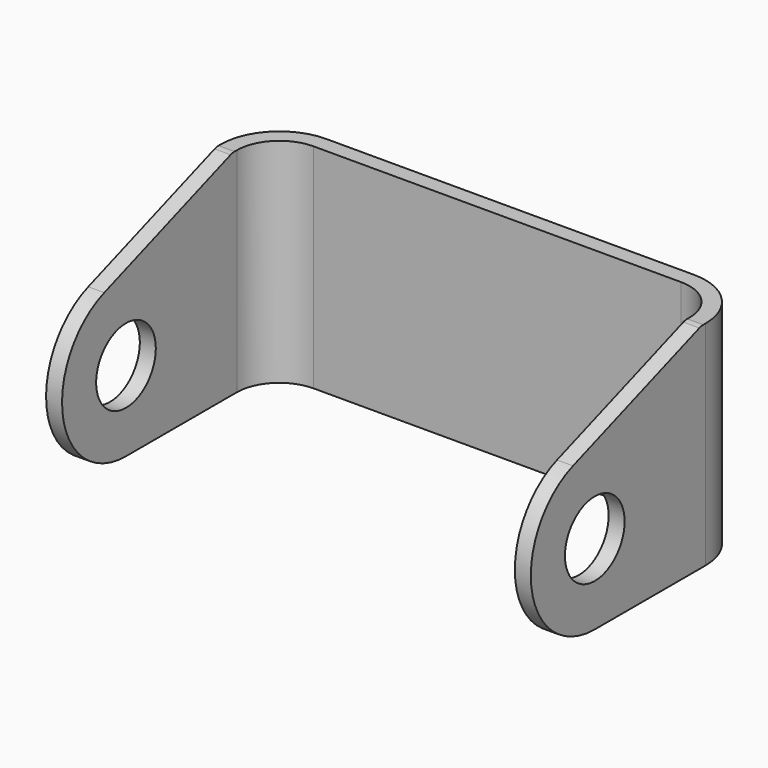
from build123d import *

# Parameters (mm, degrees)
F0_R        = 7
F1_DEPTH    = 91
F2_R        = 11
F3_T        = -3
F4_DEPTH    = 100
F5_T1_DEPTH = 5.6326126102
F5_T3_DEPTH = 5.6326126102


# Not quite as in the source:
# - a fillet or chamfer that OpenCascade refuses, or shapes differently, is made with other operations: its cross-section is extruded or revolved along the edge and cut away or added


with BuildPart() as f1:
    # F0 (on Right) → F1 (new body)
    with BuildSketch(Plane.YZ):
        with BuildLine():
            ThreePointArc((-5.1046863561, 14.1046863561), (8.6148042537, 12.2794603982), (15, 0))
            ThreePointArc((15, 0), (10.6066017178, -10.6066017178), (0, -15))
            Line((0, -15), (37, -15))
            Line((37, -15), (37, 25))
            Line((37, 25), (25, 25))
            Line((25, 25), (-5.1046863561, 14.1046863561))
        make_face()
        with BuildLine():
            ThreePointArc((0, -15), (10.6066017178, -10.6066017178), (15, 0))
            ThreePointArc((15, 0), (8.6148042537, 12.2794603982), (-5.1046863561, 14.1046863561))
            ThreePointArc((-5.1046863561, 14.1046863561), (-14.7744762232, -2.5913032105), (0, -15))
        make_face()
        Circle(F0_R, mode=Mode.SUBTRACT)
        Circle(F0_R)
    extrude(amount=-F1_DEPTH)

    # F2
    f2_edges = [f1.edges().sort_by_distance(p)[0] for p in [
        (0, 37, 5),
        (-91, 37, 5),
    ]]
    fillet(f2_edges, radius=F2_R)

    # F3
    f3_openings = [f1.faces().sort_by_distance(p)[0] for p in [
        (-45.5, -14.774476, -2.591303),
        (-45.5, 18.248672, -15),
        (-45.5, 9.947657, 19.552343),
        (-45.5, 30.82309, 25),
    ]]
    offset(amount=F3_T, openings=f3_openings)

    # F0 (on Right) → F4 (cut)
    with BuildSketch(Plane.YZ):
        Circle(F0_R)
    extrude(amount=-F4_DEPTH, mode=Mode.SUBTRACT)

    # F5: fillet of radius 3 on 4 edges, made by hand

    # F5_s2 → F5_t1 (cut)
    with BuildSketch(Plane.YZ.offset(-4.3163063051)):
        with BuildLine():
            ThreePointArc((25.5265223701, 25.0004), (25.0078471195, 24.9552591608), (24.504768349, 24.821194021))
            Line((24.504768349, 24.821194021), (24.4025929469, 25.1035134232))
            ThreePointArc((24.4025929469, 25.1035134232), (24.6502768349, 25.1927283501), (24.8978245979, 25.2823194021))
            Line((24.8978245979, 25.2823194021), (25, 25.30024))
            ThreePointArc((25, 25.30024), (25.263261185, 25.30024), (25.5265223701, 25.30064))
            Line((25.5265223701, 25.30064), (25.5265223701, 25.0004))
        make_face()
    extrude(amount=F5_T1_DEPTH, mode=Mode.SUBTRACT)

    # F5_s4 → F5_t3 (cut)
    with BuildSketch(Plane.YZ.offset(-92.3163063051)):
        with BuildLine():
            ThreePointArc((25.5265223701, 25.0004), (25.0078471195, 24.9552591608), (24.504768349, 24.821194021))
            Line((24.504768349, 24.821194021), (24.4025929469, 25.1035134232))
            ThreePointArc((24.4025929469, 25.1035134232), (24.6502768349, 25.1927283501), (24.8978245979, 25.2823194021))
            Line((24.8978245979, 25.2823194021), (25, 25.30024))
            ThreePointArc((25, 25.30024), (25.263261185, 25.30024), (25.5265223701, 25.30064))
            Line((25.5265223701, 25.30064), (25.5265223701, 25.0004))
        make_face()
    extrude(amount=F5_T3_DEPTH, mode=Mode.SUBTRACT)


solid = f1.part
